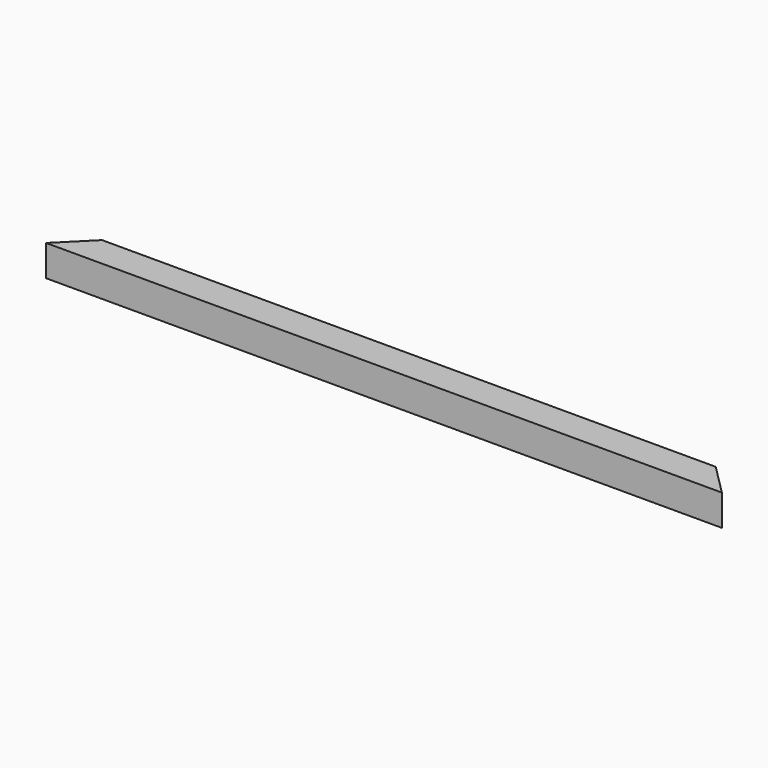
from build123d import *

# Parameters (mm, degrees)
F1_DEPTH = 1104.9
F2_SIZE2 = 50.79999
F2_SIZE  = 50.79999


# Not quite as in the source:
# - a fillet or chamfer is up to 0.001 mm smaller than in the source, because OpenCascade refuses the exact size


with BuildPart() as f1:
    # F0 (on Right) → F1 (new body)
    with BuildSketch(Plane.YZ):
        Polygon((-30.9975855052, -32.5072072446), (-24.6475855052, -32.5072072446), (-24.6475855052, 11.9427927554), (19.8024144948, 11.9427927554), (19.8024144948, 18.2927927554), (-30.9975855052, 18.2927927554), align=None)
    extrude(amount=F1_DEPTH)

    # F2 (size 50.8 and 50.8 in the source; OpenCascade refuses exactly that, so slightly less here)
    f2_edges = [f1.edges().sort_by_distance(p)[0] for p in [
        (1104.9, 19.802414, 15.117793),
        (0, 19.802414, 15.117793),
    ]]
    chamfer(f2_edges, length=F2_SIZE, length2=F2_SIZE2)


solid = f1.part
